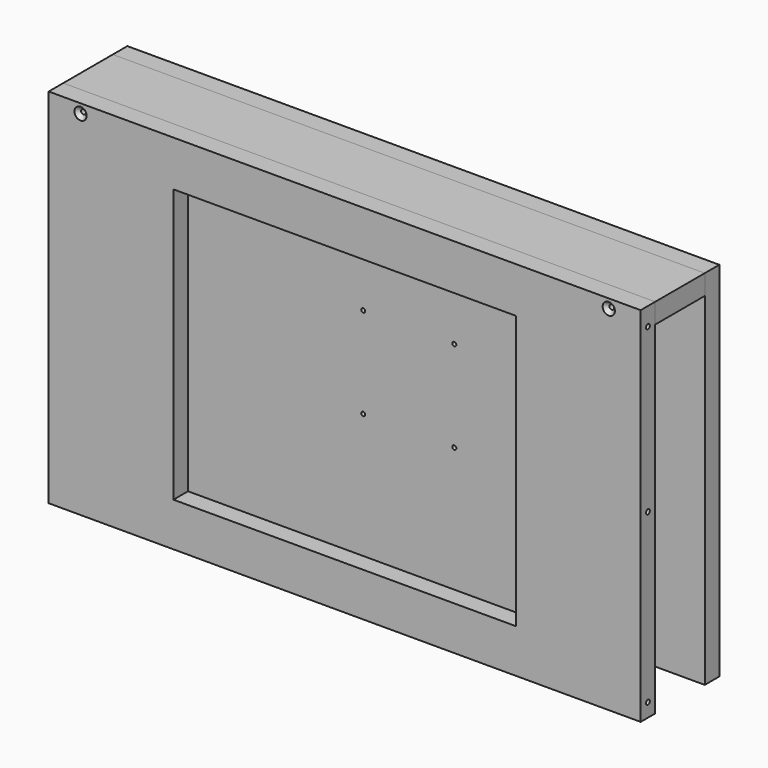
from build123d import *

# Parameters (mm, degrees)
F0_W                    = 650
F0_H                    = 398
F0_W_2                  = 376
F0_H_2                  = 300
F1_DEPTH                = 20
F4_D                    = 5.25
F4_DEPTH                = 15
F4_TIP                  = 1.5772591249
F4_ON_F3_D              = 5.25
F4_ON_F3_DEPTH          = 15
F4_ON_F3_TIP            = 1.5772591249
F5_W                    = 650
F5_H                    = 22
F6_DEPTH                = 68
F7_W                    = 650
F7_H                    = 398
F7_W_2                  = 100
F7_H_2                  = 100
F8_DEPTH                = 20
F10_D                   = 5.25
F10_DEPTH               = 40
F10_CSINK_D             = 13.44
F10_CSINK_ANGLE         = 90
F10_TIP                 = 1.5772591249
F10_2_D                 = 5.25
F10_2_DEPTH             = 40
F10_2_CSINK_D           = 13.44
F10_2_CSINK_ANGLE       = 90
F10_2_TIP               = 1.5772591249
F10_ON_F9_D             = 5.25
F10_ON_F9_DEPTH         = 40
F10_ON_F9_CSINK_D       = 13.44
F10_ON_F9_CSINK_ANGLE   = 90
F10_ON_F9_TIP           = 1.5772591249
F10_ON_F9_2_D           = 5.25
F10_ON_F9_2_DEPTH       = 40
F10_ON_F9_2_CSINK_D     = 13.44
F10_ON_F9_2_CSINK_ANGLE = 90
F10_ON_F9_2_TIP         = 1.5772591249
F11_D                   = 4.4


# Not quite as in the source:
# - a feature names something its author has since deleted; it is built from what else it names


with BuildPart() as f1:
    # F0 (on Front) → F1 (new body)
    with BuildSketch(Plane.XZ):
        Rectangle(F0_W, F0_H)
        with Locations((0, -1)):
            Rectangle(F0_W_2, F0_H_2, mode=Mode.SUBTRACT)
    extrude(amount=-F1_DEPTH)

    # F4
    with Locations(Plane(origin=(-325, 0, 0), x_dir=(0, -1, 0), z_dir=(-1, 0, 0))):
        with Locations((-10, 179), (-10, 0), (-10, -184)):
            Hole(F4_D / 2, depth=F4_DEPTH)
            with Locations((0, 0, -(F4_DEPTH + F4_TIP / 2))):  # 118° drill point
                Cone(0, F4_D / 2, F4_TIP, mode=Mode.SUBTRACT)

    # F4 on F3
    with Locations(Plane.YZ.offset(325)):
        with Locations((10, 179), (10, 0), (10, -184)):
            Hole(F4_ON_F3_D / 2, depth=F4_ON_F3_DEPTH)
            with Locations((0, 0, -(F4_ON_F3_DEPTH + F4_ON_F3_TIP / 2))):  # 118° drill point
                Cone(0, F4_ON_F3_D / 2, F4_ON_F3_TIP, mode=Mode.SUBTRACT)

    # F10
    with Locations(Plane.XZ):
        with Locations((-290, 189), (290, 189)):
            CounterSinkHole(F10_D / 2, F10_CSINK_D / 2, depth=F10_DEPTH, counter_sink_angle=F10_CSINK_ANGLE)
            with Locations((0, 0, -(F10_DEPTH + F10_TIP / 2))):  # 118° drill point
                Cone(0, F10_D / 2, F10_TIP, mode=Mode.SUBTRACT)


with BuildPart() as f6:
    # F5 (on face) → F6 (new body)
    with BuildSketch(Plane(origin=(0, 20, 0), x_dir=(-1, 0, 0), z_dir=(0, 1, 0))):
        with Locations((0, 188)):
            Rectangle(F5_W, F5_H)
    extrude(amount=F6_DEPTH)

    # F10#2
    with Locations(Plane.XZ):
        with Locations((-290, 189), (290, 189)):
            CounterSinkHole(F10_2_D / 2, F10_2_CSINK_D / 2, depth=F10_2_DEPTH, counter_sink_angle=F10_2_CSINK_ANGLE)
            with Locations((0, 0, -(F10_2_DEPTH + F10_2_TIP / 2))):  # 118° drill point
                Cone(0, F10_2_D / 2, F10_2_TIP, mode=Mode.SUBTRACT)

    # F10 on F9
    with Locations(Plane(origin=(0, 108, 0), x_dir=(-1, 0, 0), z_dir=(0, 1, 0))):
        with Locations((-225, 189), (225, 189)):
            CounterSinkHole(F10_ON_F9_D / 2, F10_ON_F9_CSINK_D / 2, depth=F10_ON_F9_DEPTH, counter_sink_angle=F10_ON_F9_CSINK_ANGLE)
            with Locations((0, 0, -(F10_ON_F9_DEPTH + F10_ON_F9_TIP / 2))):  # 118° drill point
                Cone(0, F10_ON_F9_D / 2, F10_ON_F9_TIP, mode=Mode.SUBTRACT)


with BuildPart() as f8:
    # F7 (on face) → F8 (new body)
    with BuildSketch(Plane(origin=(0, 88, 0), x_dir=(-1, 0, 0), z_dir=(0, 1, 0))):
        Rectangle(F7_W, F7_H)
        with Locations((0, -9)):
            Rectangle(F7_W_2, F7_H_2, mode=Mode.SUBTRACT)
        with Locations((0, -9)):
            Rectangle(F7_W_2, F7_H_2)
    extrude(amount=F8_DEPTH)

    # F10 on F9#2
    with Locations(Plane(origin=(0, 108, 0), x_dir=(-1, 0, 0), z_dir=(0, 1, 0))):
        with Locations((-225, 189), (225, 189)):
            CounterSinkHole(F10_ON_F9_2_D / 2, F10_ON_F9_2_CSINK_D / 2, depth=F10_ON_F9_2_DEPTH, counter_sink_angle=F10_ON_F9_2_CSINK_ANGLE)
            with Locations((0, 0, -(F10_ON_F9_2_DEPTH + F10_ON_F9_2_TIP / 2))):  # 118° drill point
                Cone(0, F10_ON_F9_2_D / 2, F10_ON_F9_2_TIP, mode=Mode.SUBTRACT)

    # F11 (through all)
    with Locations(Plane(origin=(0, 88, 0), x_dir=(-1, 0, 0), z_dir=(0, -1, 0))):
        with Locations((-50, -41), (50, -41), (50, 59), (-50, 59)):
            Hole(F11_D / 2)


solid = Compound([f1.part, f6.part, f8.part])
